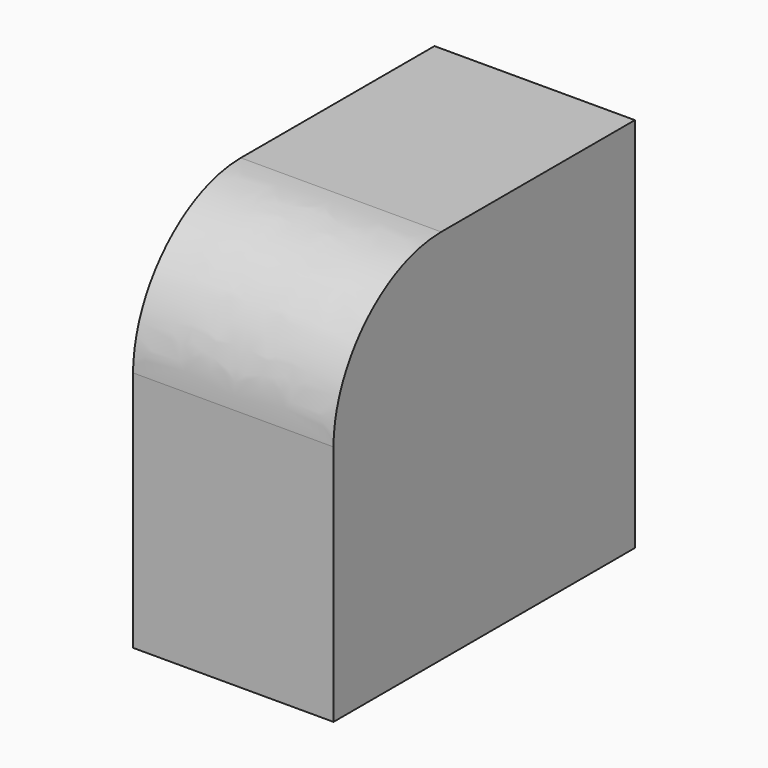
from build123d import *

# Parameters (mm, degrees)
F0_W        = 33.782
F0_H        = 63.5
F1_DEPTH    = 63.5
F2_T1_DEPTH = 147.2258952959


# Not quite as in the source:
# - a fillet or chamfer that OpenCascade refuses, or shapes differently, is made with other operations: its cross-section is extruded or revolved along the edge and cut away or added


with BuildPart() as f1:
    # F0 (on Top) → F1 (new body)
    with BuildSketch(Plane.XY):
        with Locations((-10.1092787267, 6.0263396353)):
            Rectangle(F0_W, F0_H)
    extrude(amount=F1_DEPTH)

    # F2: fillet of radius 22.6887790592 on 1 edges, made by hand

    # F2_s2 → F2_t1 (cut)
    with BuildSketch(Plane.YZ.offset(-83.7222263746)):
        with BuildLine():
            add(Edge.make_bspline(
                [(-25.7236603647, 40.8112209408), (-25.7236603647, 63.5), (-3.0348813056, 63.5)],
                knots=[0, 0, 0, 1, 1, 1], degree=2, weights=[1, 0.6666666667, 1]))
            Line((-3.0348813056, 63.5), (-25.7236603647, 63.5))
            Line((-25.7236603647, 63.5), (-25.7236603647, 40.8112209408))
        make_face()
    extrude(amount=F2_T1_DEPTH, mode=Mode.SUBTRACT)


solid = f1.part
